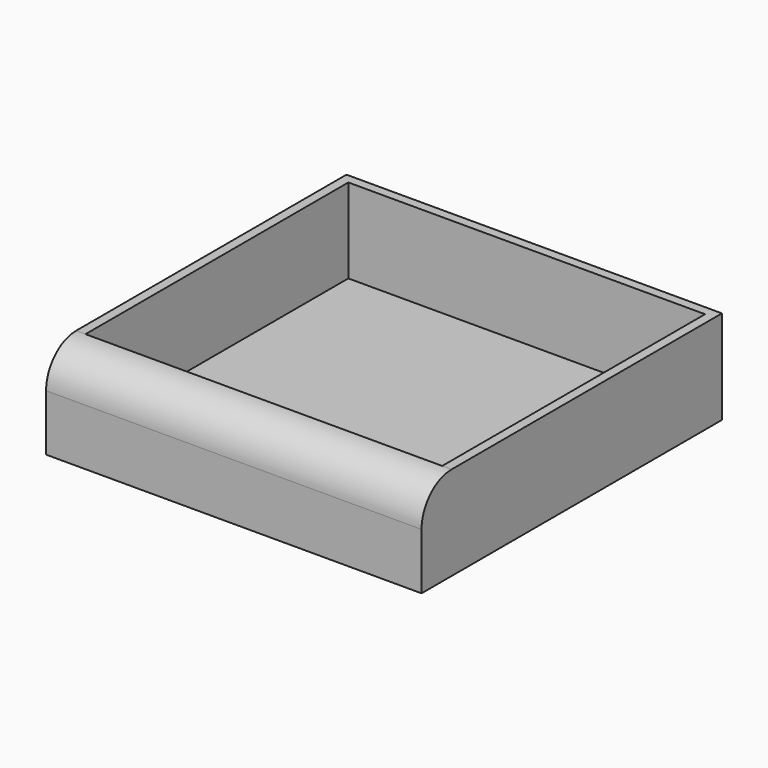
from build123d import *

# Parameters (mm, degrees)
F0_W     = 100
F0_H     = 100
F1_DEPTH = 25
F2_R     = 10
F3_T     = -2.5


# Not quite as in the source:
# - a shell that OpenCascade refuses in one call is made with other operations: the cavity is built on its own and cut out


with BuildPart() as f1:
    # F0 (on Top) → F1 (new body)
    with BuildSketch(Plane.XY):
        Rectangle(F0_W, F0_H)
    extrude(amount=F1_DEPTH)

    # F2
    f2_edges = [f1.edges().sort_by_distance(p)[0] for p in [
        (0, -50, 25),
    ]]
    fillet(f2_edges, radius=F2_R)

    # F3: a shell. OpenCascade refuses it in one call, so the cavity is built on its own and cut out:
    # the body offset inwards by the wall thickness, plus a prism from it out through each open face.
    f3_core = offset(f1.part, amount=F3_T, mode=Mode.PRIVATE)
    f3_exits = [f3_core.faces().sort_by_distance(p)[0] for p in [
        (0, 3.75, 22.5),
    ]]
    add(f3_core, mode=Mode.SUBTRACT)
    extrude(f3_exits, amount=-F3_T, mode=Mode.SUBTRACT)


solid = f1.part
